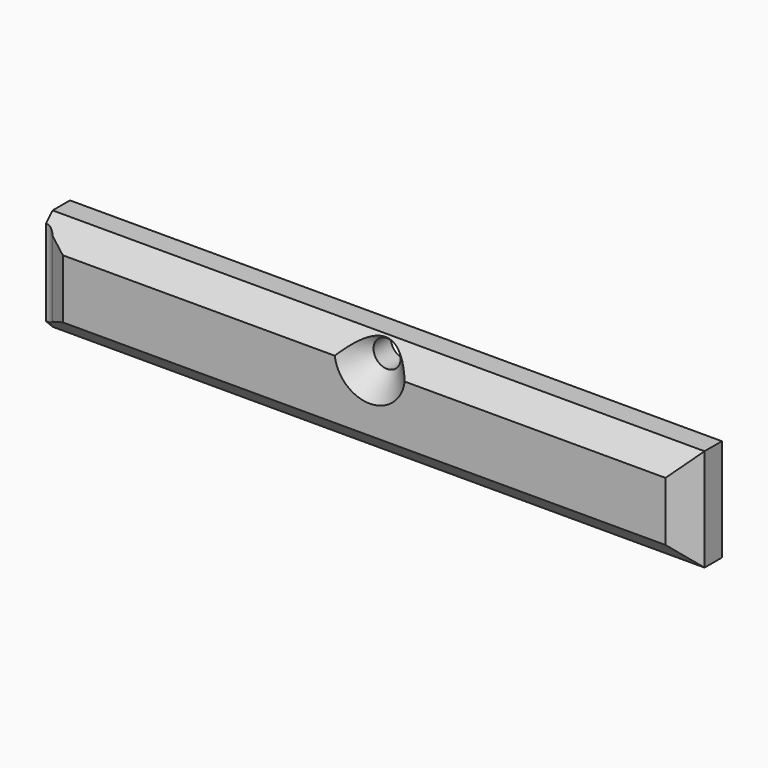
from build123d import *

# Parameters (mm, degrees)
F2_DEPTH    = 10.16
F3_D        = 6.35
F5_D        = 6.35
F6_T1_DEPTH = 175.6033201743
F6_T3_DEPTH = 41.5657076026
F6_T5_DEPTH = 50.1161940355
F7_T        = -2.54


# Not quite as in the source:
# - a fillet or chamfer that OpenCascade refuses, or shapes differently, is made with other operations: its cross-section is extruded or revolved along the edge and cut away or added


with BuildPart() as f2:
    # F0 (on Front) → F2 (new body)
    with BuildSketch(Plane.XZ):
        Polygon((75.9512782097, 0), (0, 0), (-76.6545310616, 0), (-76.6545310616, -23.9878948778), (75.9512782097, -23.9878948778), align=None)
    extrude(amount=-F2_DEPTH)

    # F3 (through all)
    with Locations(Plane.XY):
        with Locations((-76.6987428069, 0)):
            Hole(F3_D / 2)

    # F5 (through all)
    with Locations(Plane(origin=(0, 10.16, 0), x_dir=(-1, 0, 0), z_dir=(0, 1, 0))):
        with Locations((-1.640441129, -4.0405564941)):
            Hole(F5_D / 2)

    # F6: chamfer of 5.08 on 5 edges, made by hand

    # F6_s2 → F6_t1 (cut)
    with BuildSketch(Plane.YZ.offset(-86.5878923858)):
        Polygon((0, -18.9078948778), (5.08, -23.9878948778), (0, -23.9878948778), align=None)
        Polygon((5.08, 0), (0, -5.08), (0, 0), align=None)
    extrude(amount=F6_T1_DEPTH, mode=Mode.SUBTRACT)

    # F6_s4 → F6_t3 (cut)
    with BuildSketch(Plane.XY.offset(-32.7768012402)):
        with BuildLine():
            Line((-70.1919290705, 0), (-74.1961221391, 1.9538461538))
            ThreePointArc((-74.1961221391, 1.9538461538), (-73.722763255, 1.1064224811), (-73.5237428069, 0))
            Line((-73.5237428069, 0), (-70.1919290705, 0))
        make_face()
    extrude(amount=F6_T3_DEPTH, mode=Mode.SUBTRACT)

    # F6_s6 → F6_t5 (cut)
    with BuildSketch(Plane.XY.offset(-37.0520444567)):
        Polygon((70.8712782097, 0), (75.9512782097, 5.08), (75.9512782097, 0), align=None)
    extrude(amount=F6_T5_DEPTH, mode=Mode.SUBTRACT)

    # F6_s7 → F6_t8 (revolve, cut)
    with BuildSketch(Plane.XY.offset(-4.0405564941)):
        Polygon((-6.614558871, 0), (-1.534558871, 5.08), (-1.534558871, 0), align=None)
    revolve(axis=Axis((1.640441129, 0, -4.0405564941), (0, 1, 0)), mode=Mode.SUBTRACT)

    # F7
    f7_openings = [f2.faces().sort_by_distance(p)[0] for p in [
        (-0.369011, 10.16, -12.063354),
    ]]
    offset(amount=F7_T, openings=f7_openings)


solid = f2.part
